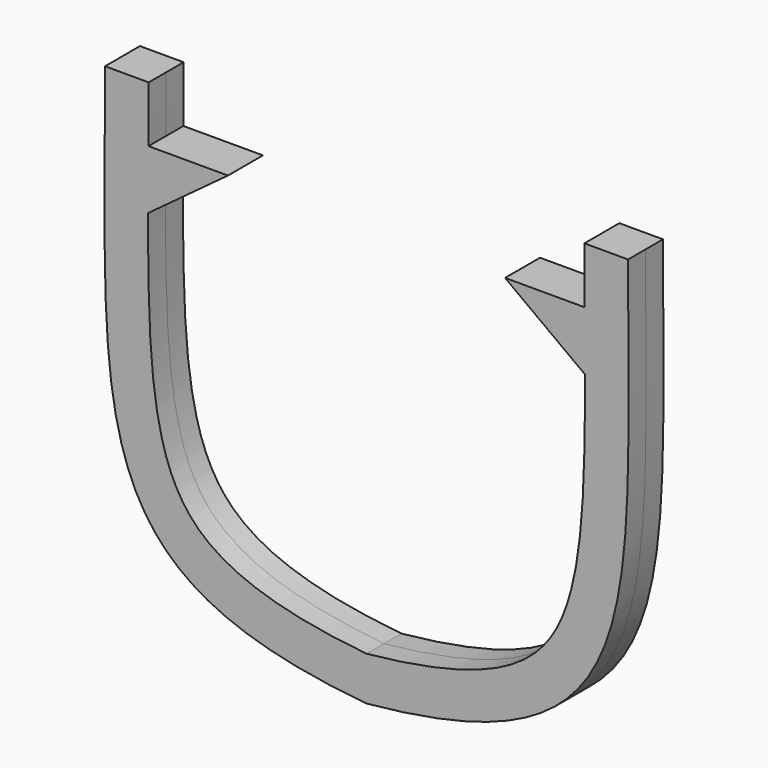
from build123d import *

# Parameters (mm, degrees)
F1_DEPTH = 5


# Not quite as in the source:
# - ends of sketch curves that miss each other by under 0.0002 mm in the source are joined
# - the dataset's text gives a spline's control points without its knots; the knots are read off the source's solid


with BuildPart() as f1:
    # F0 (on Front) → F1 (new body, symmetric)
    with BuildSketch(Plane.XZ):
        with BuildLine():
            add(Edge.make_bspline(
                [(0, 0), (-65.4905810952, 6.1836594649), (-59.8874362842, 35.6965847313), (-59.8874362842, 109)],
                knots=[0, 0, 0, 0, 124.3684245486, 124.3684245486, 124.3684245486, 124.3684245486], degree=3))
            Line((0, 0), (0, 10.0466714589))
            add(Edge.make_bspline(
                [(0, 10.0466714589), (-3.5441174674, 10.3979528849), (-10.4084893537, 11.2783893872), (-19.2104738807, 13.0740190821), (-26.578945278, 15.3681181657), (-32.3879548596, 18.0402600919), (-36.8465048652, 21.0201088718), (-40.2781462463, 24.3295586003), (-43.0206977549, 28.1637605079), (-45.2679587147, 32.8088657303), (-47.0604635141, 38.4745167968), (-48.3934054984, 45.2449692868), (-49.2866010119, 53.1289585403), (-49.9546159991, 64.8835298112), (-50.021972749, 75.185723257), (-50.0028210201, 82.629999345)],
                knots=[0.0050473797, 0.0050473797, 0.0050473797, 0.0050473797, 0.0625, 0.125, 0.1875, 0.25, 0.3125, 0.375, 0.4375, 0.5, 0.5625, 0.625, 0.6875, 0.75, 0.8703716807, 0.8703716807, 0.8703716807, 0.8703716807], degree=3))
            add(Edge.make_bspline(
                [(-50.0028210201, 82.629999345), (-50.0020846316, 82.9162335063), (-49.9896693865, 87.2111277909), (-49.9578295544, 91.7251611462), (-49.9320982819, 96.1299997307)],
                knots=[0.8703716807, 0.8703716807, 0.8703716807, 0.8703716807, 0.875, 0.9395817876, 0.9395817876, 0.9395817876, 0.9395817876], degree=3))
            add(Edge.make_bspline(
                [(-49.9320982819, 96.1299997307), (-49.9080263988, 100.2507737451), (-49.8874371385, 104.5401725024), (-49.8874362842, 108.9997224321)],
                knots=[0.9395817876, 0.9395817876, 0.9395817876, 0.9395817876, 0.9999987465, 0.9999987465, 0.9999987465, 0.9999987465], degree=3))
            Line((-49.8874362842, 108.9997224321), (-59.8874362842, 109))
        make_face()
        with BuildLine():
            Line((0, 10.0466714589), (0, 0))
            add(Edge.make_bspline(
                [(0, 0), (65.4905810952, 6.1836594649), (59.8874362842, 35.6965847313), (59.8874362842, 109)],
                knots=[0, 0, 0, 0, 124.3684245486, 124.3684245486, 124.3684245486, 124.3684245486], degree=3))
            Line((59.8874362842, 109), (49.8874362842, 109))
            add(Edge.make_bspline(
                [(49.9320982819, 96.1299997307), (49.9080258994, 100.2508592391), (49.8874362842, 104.5403504874), (49.8874362842, 109)],
                knots=[0.9395817876, 0.9395817876, 0.9395817876, 0.9395817876, 1, 1, 1, 1], degree=3))
            add(Edge.make_bspline(
                [(50.0028210201, 82.629999345), (50.0020846316, 82.9162335063), (49.9896693865, 87.2111277909), (49.9578295544, 91.7251611462), (49.9320982819, 96.1299997307)],
                knots=[0.8703716807, 0.8703716807, 0.8703716807, 0.8703716807, 0.875, 0.9395817876, 0.9395817876, 0.9395817876, 0.9395817876], degree=3))
            add(Edge.make_bspline(
                [(0, 10.0466714589), (3.5441174674, 10.3979528849), (10.4084893537, 11.2783893872), (19.2104738807, 13.0740190821), (26.578945278, 15.3681181657), (32.3879548596, 18.0402600919), (36.8465048652, 21.0201088718), (40.2781462463, 24.3295586003), (43.0206977549, 28.1637605079), (45.2679587147, 32.8088657303), (47.0604635141, 38.4745167968), (48.3934054984, 45.2449692868), (49.2866010119, 53.1289585403), (49.9546159991, 64.8835298112), (50.021972749, 75.185723257), (50.0028210201, 82.629999345)],
                knots=[0.0050473797, 0.0050473797, 0.0050473797, 0.0050473797, 0.0625, 0.125, 0.1875, 0.25, 0.3125, 0.375, 0.4375, 0.5, 0.5625, 0.625, 0.6875, 0.75, 0.8703716807, 0.8703716807, 0.8703716807, 0.8703716807], degree=3))
        make_face()
        with BuildLine():
            add(Edge.make_bspline(
                [(-50.0028210201, 82.629999345), (-50.0020846316, 82.9162335063), (-49.9896693865, 87.2111277909), (-49.9578295544, 91.7251611462), (-49.9320982819, 96.1299997307)],
                knots=[0.8703716807, 0.8703716807, 0.8703716807, 0.8703716807, 0.875, 0.9395817876, 0.9395817876, 0.9395817876, 0.9395817876], degree=3))
            Line((-50.0028210201, 82.629999345), (-31.7220522796, 96.1299994619))
            Line((-31.7220522796, 96.1299994619), (-49.9320982819, 96.1299997307))
        make_face()
        with BuildLine():
            Line((31.7220522796, 96.1299994619), (50.0028664554, 82.6299994619))
            add(Edge.make_bspline(
                [(50.0028664554, 82.6299994619), (50.0020846316, 82.9162335063), (49.9896693865, 87.2111277909), (49.9578295544, 91.7251611462), (49.9320982819, 96.1299997307)],
                knots=[0.8703716807, 0.8703716807, 0.8703716807, 0.8703716807, 0.875, 0.9395817876, 0.9395817876, 0.9395817876, 0.9395817876], degree=3))
            Line((49.9320982819, 96.1299997307), (31.7220522796, 96.1299994619))
        make_face()
    extrude(amount=F1_DEPTH, both=True)


solid = f1.part
